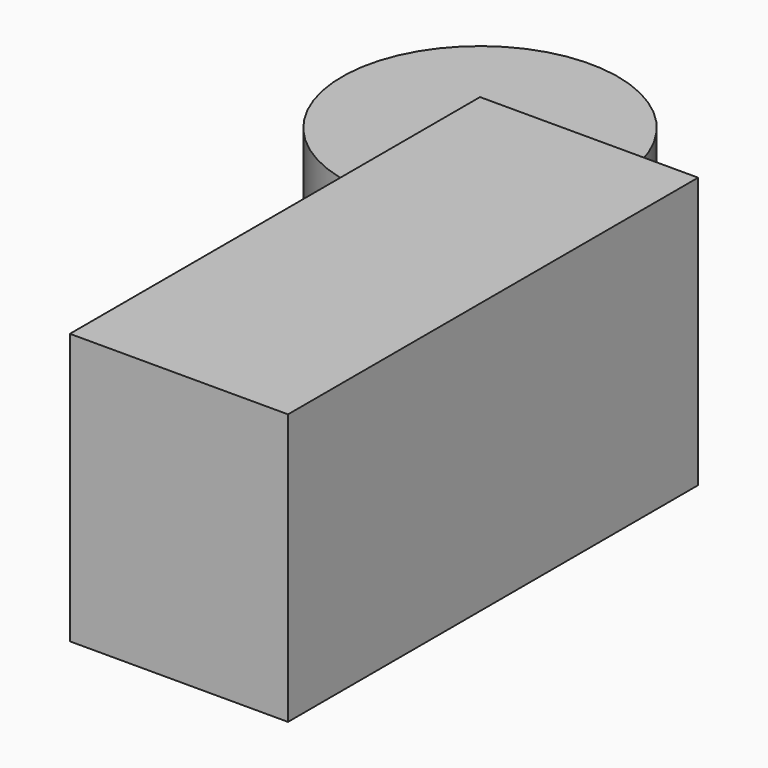
from build123d import *

# Parameters (mm, degrees)
F0_R     = 28.0405076849
F1_DEPTH = 49.53
F2_W     = 44.3078614771
F2_H     = 55.0068765879
F3_DEPTH = 104.14


with BuildPart() as f1:
    # F0 (on Top) → F1 (new body)
    with BuildSketch(Plane.XY):
        Circle(F0_R)
    extrude(amount=F1_DEPTH)

    # F2 (on Front) → F3 (join)
    with BuildSketch(Plane.XZ):
        with Locations((22.1539307386, 27.5034382939)):
            Rectangle(F2_W, F2_H)
    extrude(amount=F3_DEPTH)


solid = f1.part
